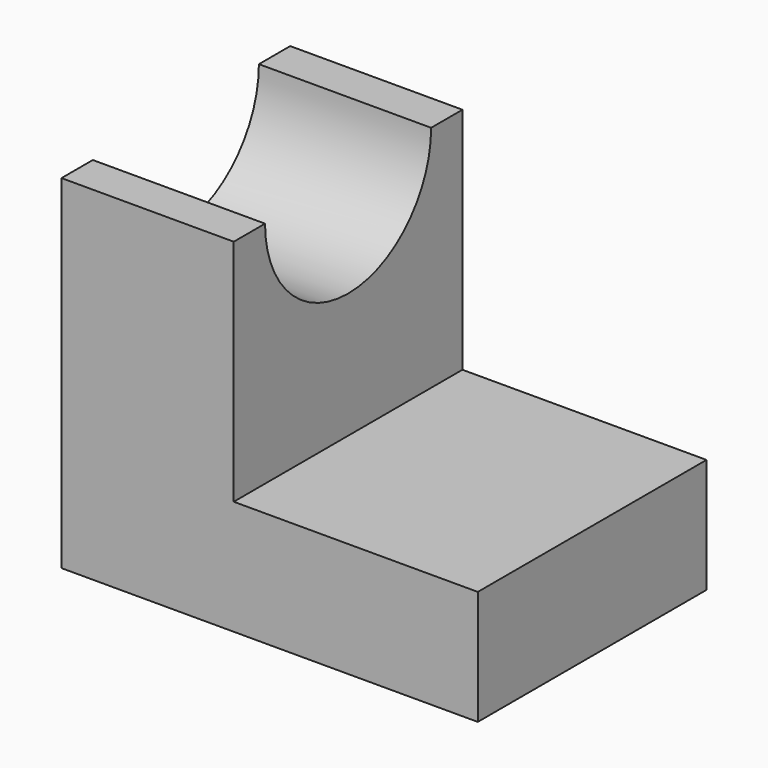
from build123d import *

# Parameters (mm, degrees)
F0_W     = 92.3780202866
F0_H     = 63.4378064424
F1_DEPTH = 25.4
F2_W     = 38.2190011442
F2_H     = 63.4378064424
F3_DEPTH = 50.8
F7_DEPTH = 50.8


# Not quite as in the source:
# - the program builds the solid bodies; features that only make, move or delete a surface that nothing else refers to are left out


with BuildPart() as f1:
    # F0 (on Top) → F1 (new body)
    with BuildSketch(Plane.XY):
        with Locations((-0.0018253922, 5.7058585808)):
            Rectangle(F0_W, F0_H)
    extrude(amount=F1_DEPTH)

    # F2 (on face) → F3 (join)
    with BuildSketch(Plane.XY.offset(25.4)):
        with Locations((-27.0813349634, 5.7058585808)):
            Rectangle(F2_W, F2_H)
    extrude(amount=F3_DEPTH)

    # F6 (on face) → F7 (cut)
    with BuildSketch(Plane.YZ.offset(-7.9718343914)):
        with BuildLine():
            ThreePointArc((-17.3291587886, 76.2), (5.7058585808, 53.1649826306), (28.7408759501, 76.2))
            Line((28.7408759501, 76.2), (-17.3291587886, 76.2))
        make_face()
    extrude(amount=-F7_DEPTH, mode=Mode.SUBTRACT)


solid = f1.part
